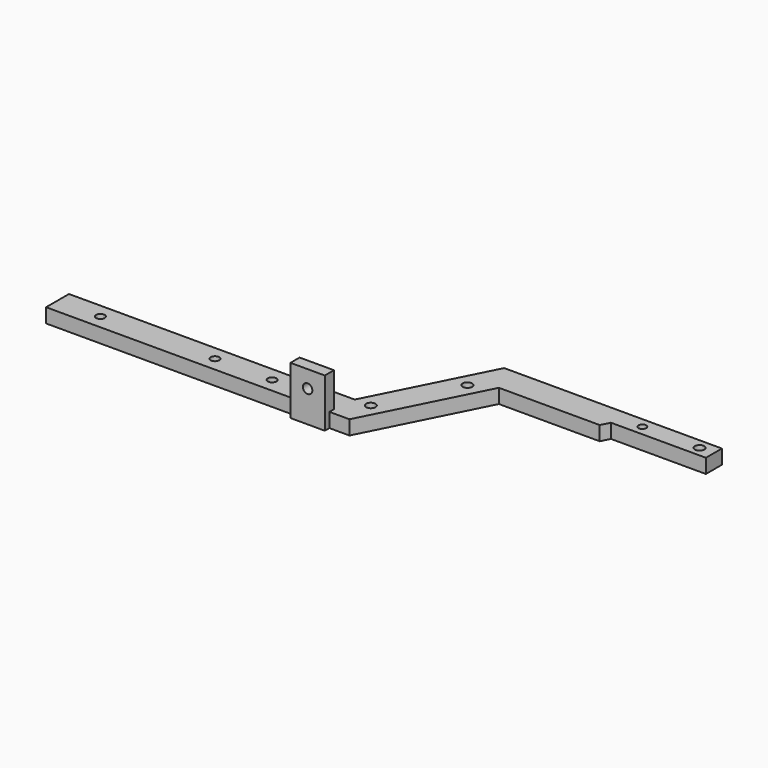
from build123d import *

# Parameters (mm, degrees)
F0_R     = 1.5
F1_DEPTH = 5
F2_DEPTH = 268
F3_R     = 1.65
F3_R_2   = 1.35
F4_DEPTH = 5.001
F5_W     = 12
F5_H     = 2
F6_DEPTH = 12
F7_DEPTH = 5
F8_R     = 1.65
F9_DEPTH = 52.0010001044


# Not quite as in the source:
# - an extrude ends at something that could not be found from the text; its depth is read off the source's solid


with BuildPart() as f1:
    # F0 (on Top) → F1 (new body)
    with BuildSketch(Plane.XY):
        Polygon((-52.0408339798, -45.9276453106), (-151.9144345724, -45.9276453106), (-151.9144345724, -55.9276454151), (-45.8887560524, -55.9276454151), (-25.683571109, -15.9276453106), (9.5701563833, -15.9276453106), (11.0855654276, -12.9276453106), (44.264588505, -12.9276453106), (44.264588505, -5.9276453106), (27.9570557177, -5.9276453106), (-31.8356490892, -5.9276453106), (-31.9144345724, -6.0836161342), align=None)
        with Locations((-136.9144345724, -50.9276454151)):
            Circle(F0_R, mode=Mode.SUBTRACT)
        with Locations((-96.9144345724, -50.9276454151)):
            Circle(F0_R, mode=Mode.SUBTRACT)
        with Locations((-76.9144345724, -50.9276454151)):
            Circle(F0_R, mode=Mode.SUBTRACT)
    extrude(amount=F1_DEPTH)

    # F0 (on Top) → F2 (cut, through all)
    with BuildSketch(Plane.XY):
        with Locations((-76.9144345724, -50.9276454151)):
            Circle(F0_R)
        with Locations((-96.9144345724, -50.9276454151)):
            Circle(F0_R)
    extrude(amount=-F2_DEPTH, mode=Mode.SUBTRACT)

    # F3 (on face) → F4 (cut, through all)
    with BuildSketch(Plane.XY.offset(5)):
        with Locations((39.264588505, -9.4276453106)):
            Circle(F3_R)
        with Locations((19.264588505, -9.4276453106)):
            Circle(F3_R_2)
        with Locations((-33.3638369572, -20.042586615)):
            Circle(F3_R)
        with Locations((-46.4391469312, -45.9276454151)):
            Circle(F3_R)
    extrude(amount=-F4_DEPTH, mode=Mode.SUBTRACT)

    # F5 (on face) → F6 (join)
    with BuildSketch(Plane.XY.offset(5)):
        with Locations((-58.9144345724, -54.9276454151)):
            Rectangle(F5_W, F5_H)
        with Locations((-58.9144345724, -56.9276454151)):
            Rectangle(F5_W, F5_H)
    extrude(amount=F6_DEPTH)

    # F7 (add): a face of the model
    f7_faces = [f1.faces().sort_by_distance(p)[0] for p in [
        (-58.9144345724, -56.9276454151, 5),
    ]]
    extrude(f7_faces, amount=F7_DEPTH)

    # F8 (on face) → F9 (cut, through all)
    with BuildSketch(Plane.XZ.offset(57.9276454151)):
        with Locations((-58.9144345724, 11)):
            Circle(F8_R)
    extrude(amount=-F9_DEPTH, mode=Mode.SUBTRACT)


solid = f1.part
